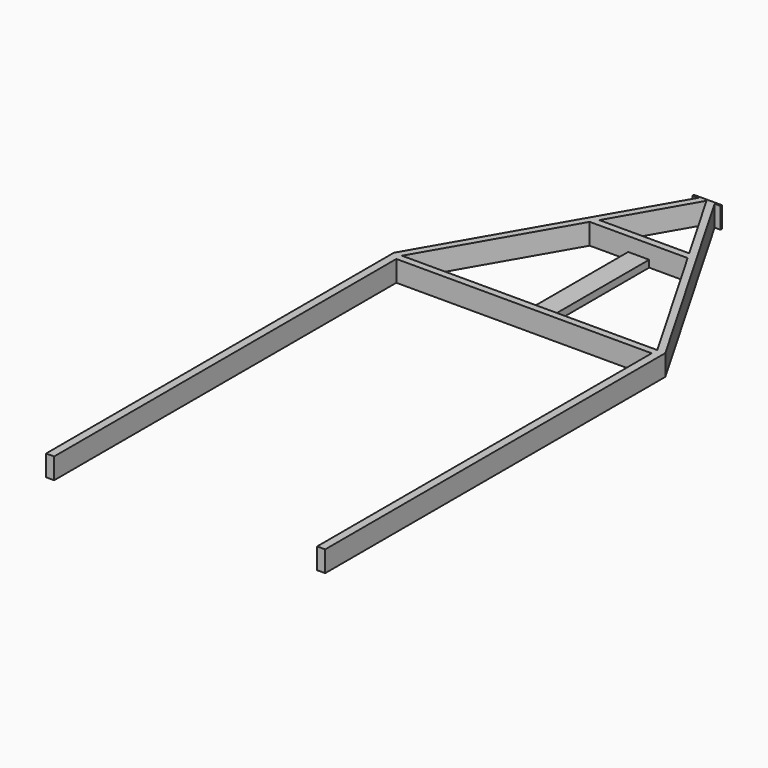
from build123d import *

# Parameters (mm, degrees)
F0_R     = 53.975
F1_DEPTH = 152.4
F2_W     = 152.4
F2_H     = 989.8670365256
F3_DEPTH = 101.6
F6_DEPTH = 2540
F7_DEPTH = 2540


# Not quite as in the source:
# - the program builds the solid bodies; features that only make, move or delete a surface that nothing else refers to are left out


with BuildPart() as f1:
    # F0 (on Top) → F1 (new body)
    with BuildSketch(Plane.XY):
        Polygon((-864.3519468606, 152.9725746632), (-864.3519468606, 203.7725746632), (-923.0107342102, 203.7725746632), (-923.0107342102, -412.8196537495), (-864.3519468606, -412.8196537495), align=None)
        Polygon((989.8480531394, 203.7725746632), (989.8480531394, 152.9725746632), (989.8480531394, -343.7095284462), (1048.5068404891, -343.7095284462), (1048.5068404891, 203.7725746632), align=None)
        Polygon((121.4068404891, 1809.5568783603), (62.7480531394, 1809.5568783603), (389.0186594646, 1244.4396111888), (418.3480531394, 1193.6396111888), (989.8480531394, 203.7725746632), (1048.5068404891, 203.7725746632), align=None)
        Polygon((-263.5225531857, 1244.4396111888), (-292.8519468606, 1193.6396111888), (-36.2017042935, 1193.6396111888), (-13.4519468606, 1193.6396111888), (116.1982957065, 1193.6396111888), (138.9480531394, 1193.6396111888), (418.3480531394, 1193.6396111888), (389.0186594646, 1244.4396111888), align=None)
        Polygon((-13.4519468606, 203.7725746632), (-864.3519468606, 203.7725746632), (-864.3519468606, 152.9725746632), (989.8480531394, 152.9725746632), (989.8480531394, 203.7725746632), (138.9480531394, 203.7725746632), (62.7480531394, 203.7725746632), align=None)
        Polygon((-13.4519468606, 1193.6396111888), (-13.4519468606, 203.7725746632), (62.7480531394, 203.7725746632), (138.9480531394, 203.7725746632), (138.9480531394, 1193.6396111888), (116.1982957065, 1193.6396111888), align=None)
        with Locations((62.7480531394, 698.6915746632)):
            Circle(F0_R, mode=Mode.SUBTRACT)
        Polygon((-923.0107342102, 203.7725746632), (-864.3519468606, 203.7725746632), (-292.8519468606, 1193.6396111888), (-263.5225531857, 1244.4396111888), (62.7480531394, 1809.5568783603), (4.0892657898, 1809.5568783603), align=None)
        with Locations((62.7480531394, 698.6915746632)):
            Circle(F0_R)
        Polygon((-38.8519468606, 1809.5568783603), (4.0892657898, 1809.5568783603), (62.7480531394, 1809.5568783603), (121.4068404891, 1809.5568783603), (164.3480531394, 1809.5568783603), (164.3480531394, 1822.2568783603), (-38.8519468606, 1822.2568783603), align=None)
    extrude(amount=-F1_DEPTH)

    # F2 (on face) → F3 (cut)
    with BuildSketch(Plane.XY):
        with Locations((62.7480531394, 698.706092926)):
            Rectangle(F2_W, F2_H)
    extrude(amount=-F3_DEPTH, mode=Mode.SUBTRACT)

    # F6 (add): a face of the model
    f6_faces = [f1.faces().sort_by_distance(p)[0] for p in [
        (1019.1774468143, -343.7095284462, -76.2),
    ]]
    extrude(f6_faces, amount=F6_DEPTH)

    # F7 (add): a face of the model
    f7_faces = [f1.faces().sort_by_distance(p)[0] for p in [
        (-893.6813405354, -412.8196537495, -76.2),
    ]]
    extrude(f7_faces, amount=F7_DEPTH)


solid = f1.part
